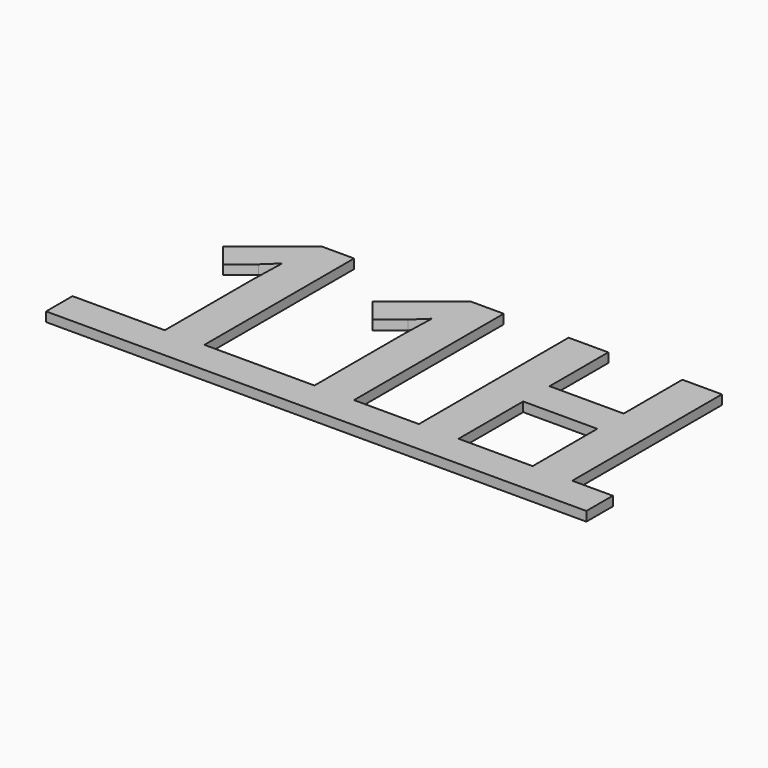
from build123d import *

# Parameters (mm, degrees)
F0_TEXT_SIZE = 1411.1111111111
F1_DEPTH     = 50.8


# Not quite as in the source:
# - a feature names something its author has since deleted; it is built from what else it names
# - Text() gives the source's letters only with a copy of the font that has no kerning and outlines rounded to 1/6400 em; it was checked with that copy


with BuildPart() as f1:
    # F0 (on Top) → F1 (new body)
    with BuildSketch(Plane.XY):
        Polygon((-177.4807680845, 0), (-177.4807680845, -177.8), (2731.1720096933, -177.8), (2731.1720096933, 0), (2512.6702735821, 0), (2299.6806902488, 0), (1900.8213152488, 0), (1687.1702735821, 0), (1337.9202735821, 0), (1124.9306902488, 0), (532.4845096933, 0), (319.4949263599, 0), align=None)
        with Locations((-50.4807680845, 0)):
            Text('11H', F0_TEXT_SIZE, font='Open Sans', font_style=FontStyle.BOLD, text_align=(TextAlign.LEFT, TextAlign.BOTTOM))
    extrude(amount=F1_DEPTH)


solid = f1.part
